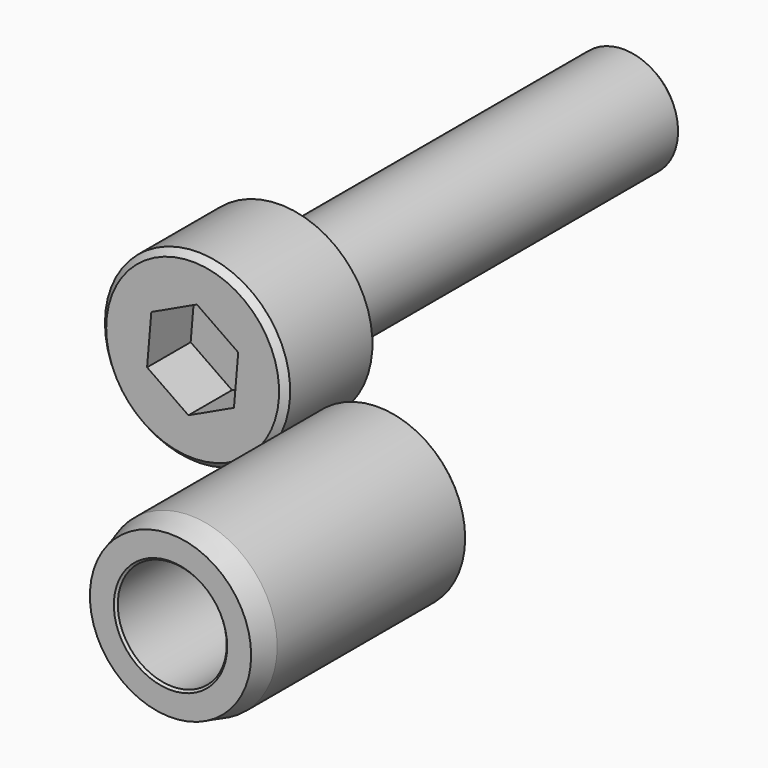
from build123d import *

# Parameters (mm, degrees)
F3_DEPTH = 2.5
F4_R     = 4
F4_R_2   = 2.5
F5_DEPTH = 12
F6_SIZE2 = 1.1196152423
F6_SIZE  = 0.3
F7_SIZE  = 0.1


with BuildPart() as f1:
    # F0 (on Top) → F1 (revolve)
    with BuildSketch(Plane.XY):
        Polygon((4.8000001721, 9.1000000201), (3.0500001721, 9.1000000201), (3.0500001721, 4.3828427326), (3.3328428846, 4.1000000201), (7.3000001721, 4.1000000201), (7.3000001721, 9.1000000201), (7.3000001721, 29.1000000201), (5.0828428846, 29.1000000201), (4.8000001721, 28.8171573076), align=None)
    revolve(axis=Axis((7.3000001721, 19.1000000201, 0), (0, 1, 0)))

    # F2 (on face) → F3 (cut)
    with BuildSketch(Plane.XZ.offset(-4.1000000201)):
        Polygon((9.390368806, 0.9816783118), (7.4950261327, 2.3011514961), (5.4046574988, 1.3194731844), (5.2096315382, -0.9816783118), (7.1049742115, -2.3011514961), (9.1953428454, -1.3194731844), align=None)
    extrude(amount=-F3_DEPTH, mode=Mode.SUBTRACT)


with BuildPart() as f5:
    # F4 (on Front) → F5 (new body)
    with BuildSketch(Plane.XZ):
        with Locations((19.1643424332, -0.3313947527)):
            Circle(F4_R)
        with Locations((19.1643424332, -0.3313947527)):
            Circle(F4_R_2, mode=Mode.SUBTRACT)
    extrude(amount=F5_DEPTH)

    # F6
    f6_edges = [f5.edges().sort_by_distance(p)[0] for p in [
        (15.164342, -12, -0.331395),
    ]]
    f6_side = f5.faces().sort_by_distance((15.27748, -12, -0.331395))[0]
    chamfer(f6_edges, length=F6_SIZE, length2=F6_SIZE2, reference=f6_side)

    # F7
    f7_edges = [f5.edges().sort_by_distance(p)[0] for p in [
        (15.164342, 0, -0.331395),
        (16.664342, 0, -0.331395),
        (16.664342, -12, -0.331395),
    ]]
    chamfer(f7_edges, length=F7_SIZE)


solid = Compound([f1.part, f5.part])
